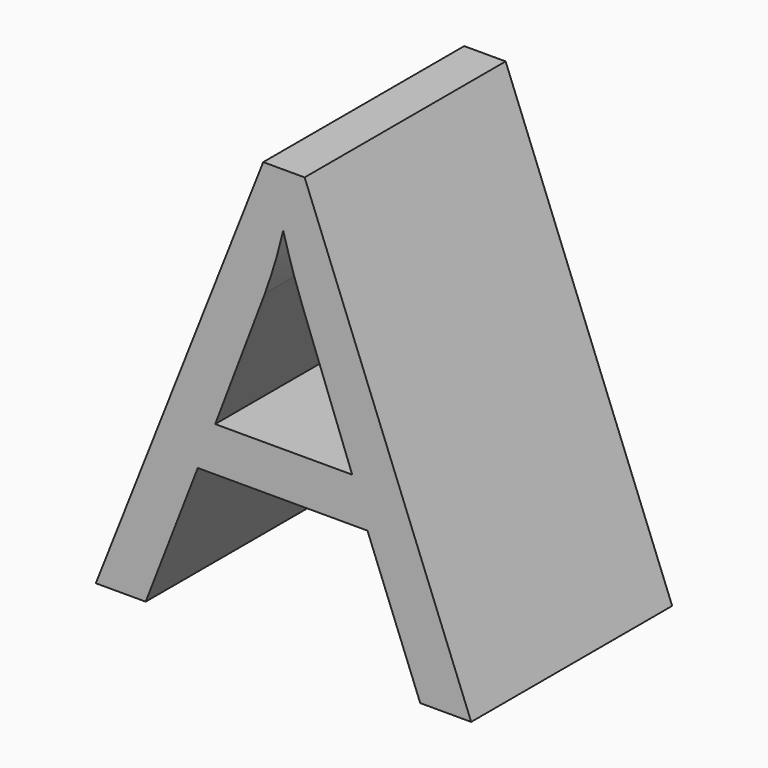
from build123d import *

# Parameters (mm, degrees)
F0_TEXT_SIZE = 59.9657107765
F1_DEPTH     = 25.4


# Not quite as in the source:
# - Text() gives the source's letters only with a copy of the font that has no kerning and outlines rounded to 1/6400 em; it was checked with that copy


with BuildPart() as f1:
    # F0 (on Front) → F1 (new body)
    with BuildSketch(Plane.XZ):
        with Locations((-37.9470513508, 19.3019062281)):
            Text('A', F0_TEXT_SIZE, font='Open Sans', text_align=(TextAlign.LEFT, TextAlign.BOTTOM))
    extrude(amount=F1_DEPTH)


solid = f1.part
